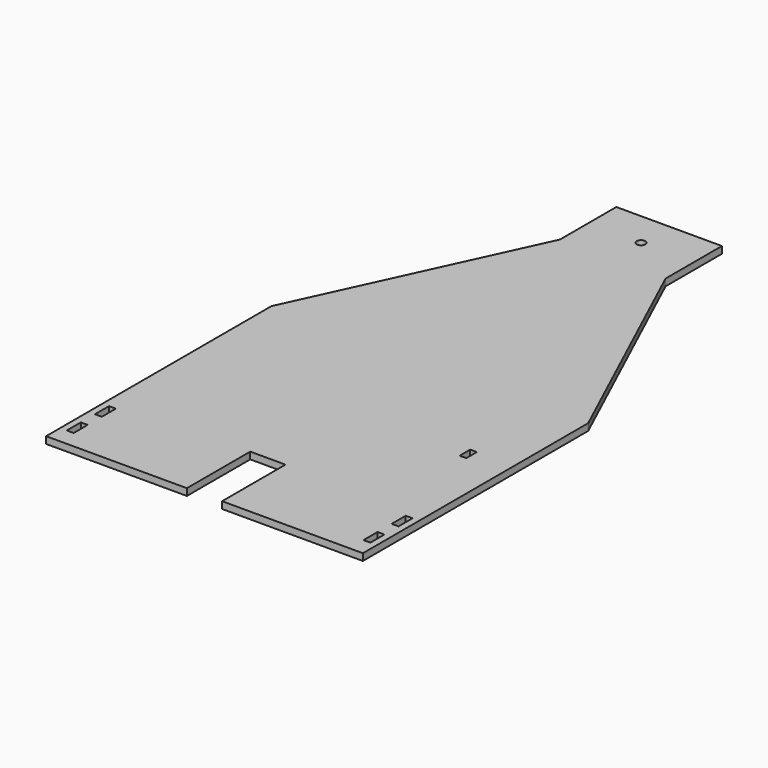
from build123d import *

# Parameters (mm, degrees)
F0_W     = 19.812
F0_H     = 50.8
F0_W_2   = 19.05
F0_H_2   = 38.1
F1_DEPTH = 19.812
F2_R     = 12.7
F3_DEPTH = 254


# Not quite as in the source:
# - a feature names something its author has since deleted; it is built from what else it names


with BuildPart() as f1:
    # F0 (on Top) → F1 (new body)
    with BuildSketch(Plane.XY):
        Polygon((-468.2972775146, 751.1484609425), (-468.2972775146, -61.6515390575), (-61.8972775146, -61.6515390575), (-61.8972775146, 166.9484609425), (39.7027224854, 166.9484609425), (39.7027224854, -61.6515390575), (446.1027224854, -61.6515390575), (446.1027224854, 751.1484609425), (141.3027224854, 1411.5484609425), (141.3027224854, 1614.7484609425), (-11.0972775146, 1614.7484609425), (-163.4972775146, 1614.7484609425), (-163.4972775146, 1411.5484609425), align=None)
        with Locations((-439.3412775146, 14.5484609425)):
            Rectangle(F0_W, F0_H, mode=Mode.SUBTRACT)
        with Locations((-439.3412775146, 116.1484609425)):
            Rectangle(F0_W, F0_H, mode=Mode.SUBTRACT)
        with Locations((417.1467224854, 14.5484609425)):
            Rectangle(F0_W, F0_H, mode=Mode.SUBTRACT)
        with Locations((417.1467224854, 116.1484609425)):
            Rectangle(F0_W, F0_H, mode=Mode.SUBTRACT)
        with Locations((328.6277224854, 465.3984609425)):
            Rectangle(F0_W_2, F0_H_2, mode=Mode.SUBTRACT)
    extrude(amount=F1_DEPTH)

    # F2 (on face) → F3 (cut)
    with BuildSketch(Plane.XY.offset(19.812)):
        with Locations((-11.0972775146, 1513.1484609425)):
            Circle(F2_R)
    extrude(amount=-F3_DEPTH, mode=Mode.SUBTRACT)


solid = f1.part
